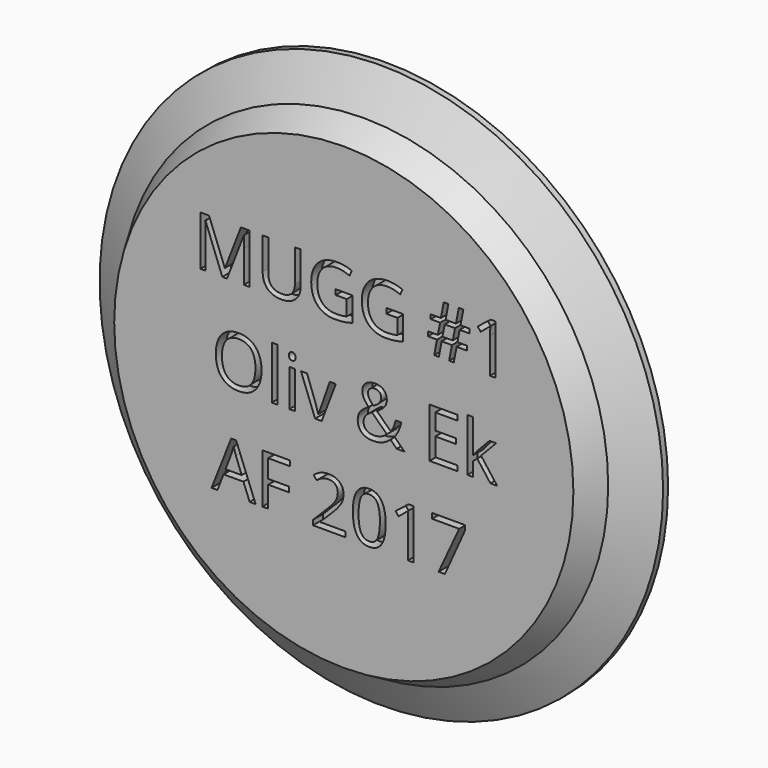
from build123d import *

# Parameters (mm, degrees)
F0_R         = 22.5
F1_DEPTH     = 6
F2_SIZE2     = 6.4951905284
F2_SIZE      = 3.75
F3_SIZE2     = 3.0310889132
F3_SIZE      = 1.75
F6_TEXT_SIZE = 5.5555555556
F7_DEPTH     = 1


# Not quite as in the source:
# - a feature names something its author has since deleted; it is built from what else it names
# - Text() gives the source's letters only with a copy of the font that has no kerning and outlines rounded to 1/6400 em; it was checked with that copy


with BuildPart() as f1:
    # F0 (on Front) → F1 (new body)
    with BuildSketch(Plane.XZ):
        Circle(F0_R)
    extrude(amount=F1_DEPTH)

    # F2
    f2_edges = [f1.edges().sort_by_distance(p)[0] for p in [
        (-22.5, -6, 0),
    ]]
    f2_side = f1.faces().sort_by_distance((-22.5, -3, 0))[0]
    chamfer(f2_edges, length=F2_SIZE, length2=F2_SIZE2, reference=f2_side)

    # F3
    f3_edges = [f1.edges().sort_by_distance(p)[0] for p in [
        (-22.5, 0, 0),
    ]]
    chamfer(f3_edges, length=F3_SIZE, length2=F3_SIZE2)

    # F4 (on Right) → F5 (revolve)
    with BuildSketch(Plane.YZ):
        Polygon((-6, 18.3349364905), (-6, 16.0048094716), (-3.9820508076, 19.5), align=None)
    revolve(axis=Axis((0, -2.9850392602, 0), (0, -1, 0)))

    # F6 (on face) → F7 (cut)
    with BuildSketch(Plane.XZ.offset(6)):
        with Locations((-12, 6)):
            Text('MUGG #1', F6_TEXT_SIZE, font='Open Sans', text_align=(TextAlign.LEFT, TextAlign.BOTTOM))
        with Locations((-10.5564236111, -1.5555555556)):
            Text('Oliv & Ek', F6_TEXT_SIZE, font='Open Sans', text_align=(TextAlign.LEFT, TextAlign.BOTTOM))
        with Locations((-10.5564236111, -9.1111111111)):
            Text('AF 2017', F6_TEXT_SIZE, font='Open Sans', text_align=(TextAlign.LEFT, TextAlign.BOTTOM))
    extrude(amount=-F7_DEPTH, mode=Mode.SUBTRACT)


solid = f1.part
